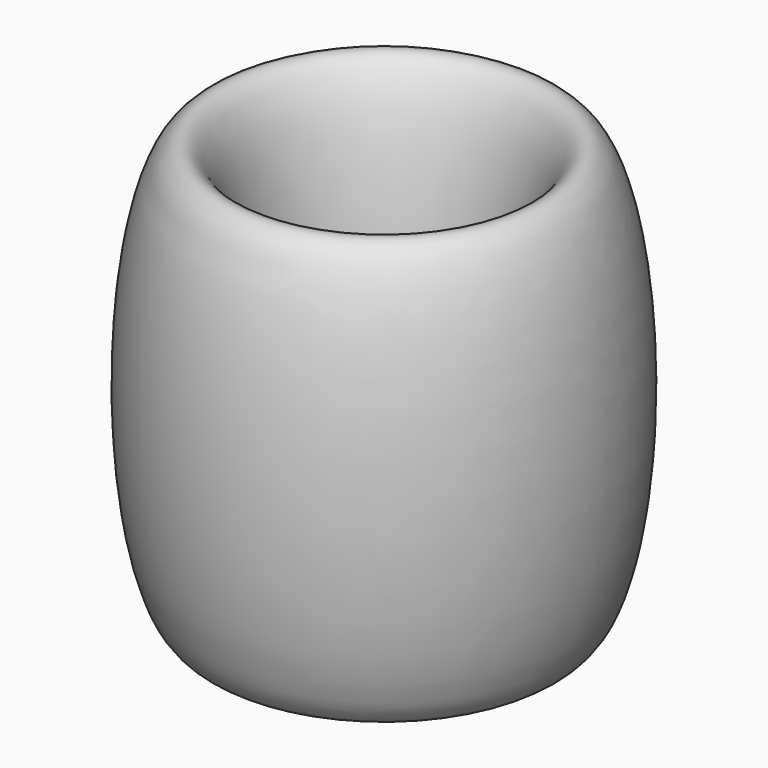
from build123d import *


# Not quite as in the source:
# - a feature names something its author has since deleted; it is built from what else it names


with BuildPart() as f1:
    # F0 (on Front) → F1 (revolve)
    with BuildSketch(Plane.XZ):
        with BuildLine():
            Line((0, 0), (18.75, 0))
            add(Edge.make_bspline(
                [(18.75, 0), (27.0192806225, 0), (24.7628117245, 31.8218415874), (22.5063428266, 63.6436831748), (15.4685240736, 46.2769981885), (8.4307053206, 28.9103132022), (14.5280449909, 6.5662935248)],
                knots=[3.1415926536, 3.1415926536, 3.1415926536, 4.9887677733, 4.9887677733, 6.8359428931, 6.8359428931, 8.6831180128, 8.6831180128, 8.6831180128], degree=2, weights=[1, 0.6029619957, 1, 0.6029619957, 1, 0.6029619957, 1]))
            ThreePointArc((14.5280449909, 6.5662935248), (13.6781742516, 2.215322721), (9.7044186209, 0.25))
            Line((9.7044186209, 0.25), (0, 0.25))
            Line((0, 0.25), (0, 0))
        make_face()
    revolve(axis=Axis((0, 0, 25), (0, 0, 1)))


solid = f1.part
